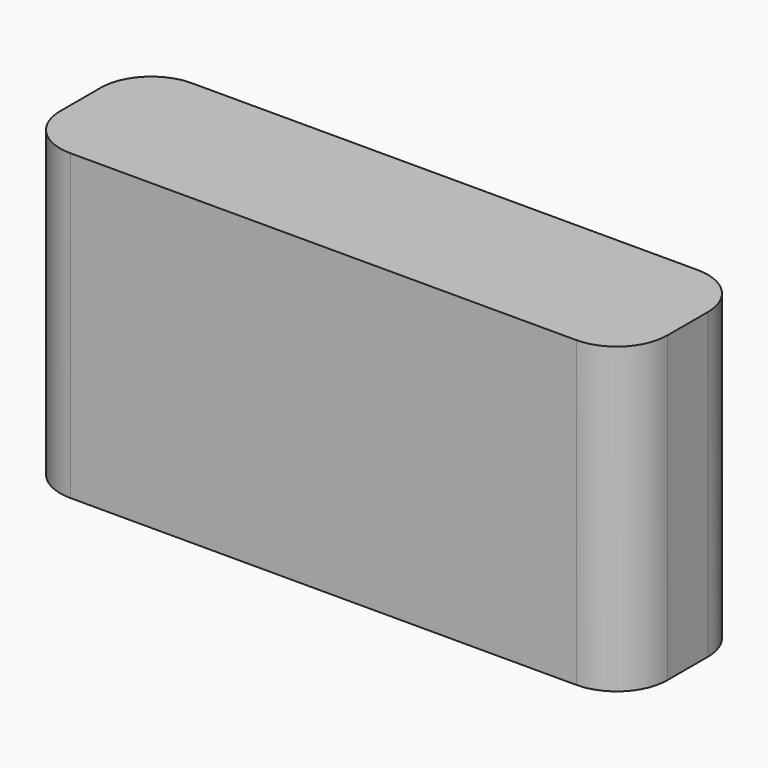
from build123d import *

# Parameters (mm, degrees)
F1_DEPTH = 30


# Not quite as in the source:
# - a feature names something its author has since deleted; it is built from what else it names


with BuildPart() as f1:
    # F0 (on Top) → F1 (new body)
    with BuildSketch(Plane.XY):
        with BuildLine():
            Line((0, -10.8138243272), (0, -5.8138243272))
            ThreePointArc((0, -5.8138243272), (-1.4644660941, -2.2782904213), (-5, -0.8138243272))
            Line((-5, -0.8138243272), (-55, -0.8138243272))
            ThreePointArc((-55, -0.8138243272), (-58.5355339059, -2.2782904213), (-60, -5.8138243272))
            Line((-60, -5.8138243272), (-60, -10.8138243272))
            ThreePointArc((-60, -10.8138243272), (-58.5355339059, -14.3493582332), (-55, -15.8138243272))
            Line((-55, -15.8138243272), (-5, -15.8138243272))
            ThreePointArc((-5, -15.8138243272), (-1.4644660941, -14.3493582332), (0, -10.8138243272))
        make_face()
    extrude(amount=F1_DEPTH)


solid = f1.part
